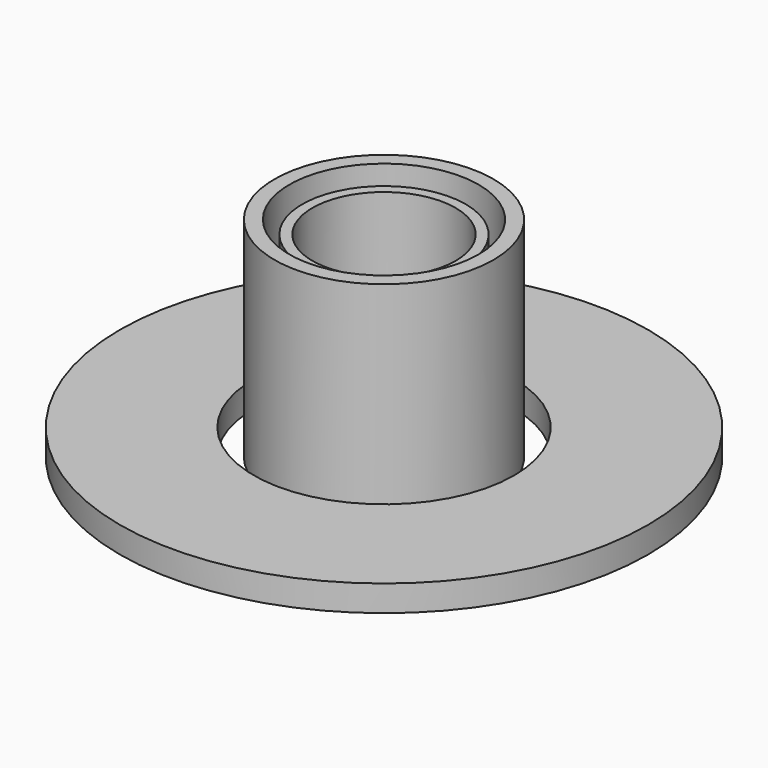
from build123d import *

# Parameters (mm, degrees)
F0_R     = 53.2061517891
F0_R_2   = 45.9801933219
F1_DEPTH = 101.6
F3_R     = 39.7127386475
F3_R_2   = 34.8221258387
F4_DEPTH = 95.25
F5_R     = 128.3623160329
F5_R_2   = 63.2849782705
F6_DEPTH = 12.7


# Not quite as in the source:
# - the program builds the solid bodies; features that only make, move or delete a surface that nothing else refers to are left out


with BuildPart() as f1:
    # F0 (on Top) → F1 (new body)
    with BuildSketch(Plane.XY):
        Circle(F0_R)
        Circle(F0_R_2, mode=Mode.SUBTRACT)
    extrude(amount=F1_DEPTH)


with BuildPart() as f4:
    # F3 (on Top) → F4 (new body)
    with BuildSketch(Plane.XY):
        Circle(F3_R)
        Circle(F3_R_2, mode=Mode.SUBTRACT)
    extrude(amount=F4_DEPTH)


with BuildPart() as f6:
    # F5 (on Top) → F6 (new body)
    with BuildSketch(Plane.XY):
        Circle(F5_R)
        Circle(F5_R_2, mode=Mode.SUBTRACT)
    extrude(amount=F6_DEPTH)


solid = Compound([f1.part, f4.part, f6.part])
